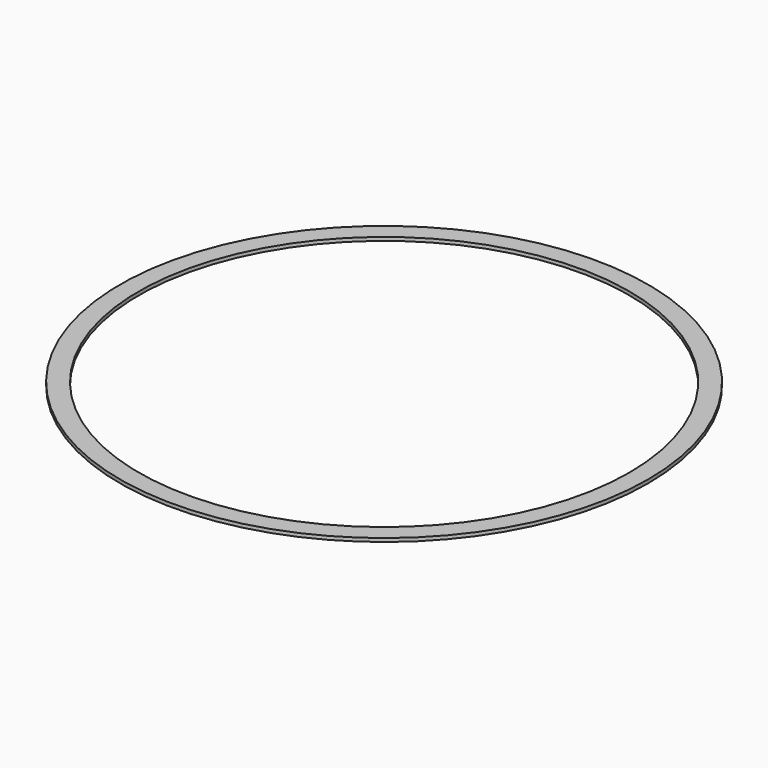
from build123d import *

# Parameters (mm, degrees)
F0_R     = 359.79227
F0_R_2   = 334.39227
F1_DEPTH = 4.7625


# Not quite as in the source:
# - a length typed as a fraction of an inch, garbled in the dataset ("3 / 203.2 mm" for 3/8 in), is restored


with BuildPart() as f1:
    # F0 (on Top) → F1 (new body)
    with BuildSketch(Plane.XY):
        Circle(F0_R)
        Circle(F0_R_2, mode=Mode.SUBTRACT)
    extrude(amount=F1_DEPTH)


solid = f1.part
